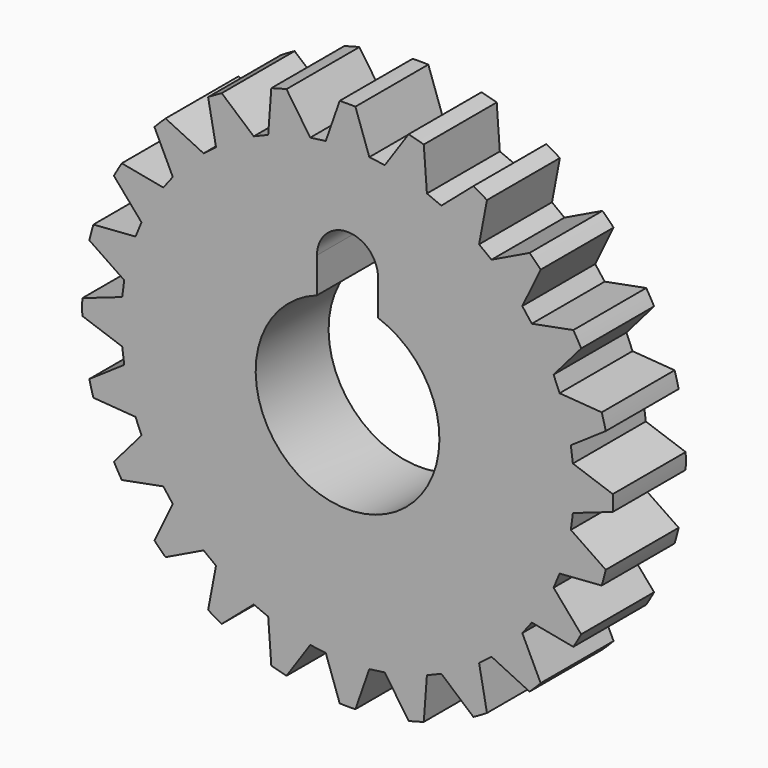
from build123d import *

# Parameters (mm, degrees)
F0_R            = 13.7922
F0_R_2          = 4.7752
F1_DEPTH        = 4.7371
F3_DEPTH        = 4.7381
F5_DEPTH        = 4.7381
F5_COPIES_COUNT = 24


# Not quite as in the source:
# - a pattern or mirror of a feature is missing from the dataset's text; its kind, count and spacing are read off the source's solid


with BuildPart() as f1:
    # F0 (on Front) → F1 (new body)
    with BuildSketch(Plane.XZ):
        Circle(F0_R)
        Circle(F0_R_2, mode=Mode.SUBTRACT)
    extrude(amount=F1_DEPTH)

    # F2 (on Front) → F3 (cut, through all)
    with BuildSketch(Plane.XZ):
        with BuildLine():
            Line((-1.5875, 6.3373), (-1.5875, 0))
            Line((-1.5875, 0), (1.5875, 0))
            Line((1.5875, 0), (1.5875, 6.3373))
            ThreePointArc((1.5875, 6.3373), (0, 7.9248), (-1.5875, 6.3373))
        make_face()
    extrude(amount=F3_DEPTH, mode=Mode.SUBTRACT)

    # F4 (on Front) → F5 (cut, through all)
    with BuildSketch(Plane.XZ):
        with BuildLine():
            Line((0.4064, 13.7922), (1.1320909341, 11.7126357032))
            Line((1.1320909341, 11.7126357032), (1.9379373174, 11.6065440142))
            Line((1.9379373174, 11.6065440142), (3.1771317781, 13.4274262413))
            ThreePointArc((3.1771317781, 13.4274262413), (1.8061892107, 13.7193691256), (0.4064, 13.7922))
        make_face()
    f5 = extrude(amount=F5_DEPTH, mode=Mode.SUBTRACT)

    # F5_copies: F5 ×24 about axis
    f5_copies_axis = Axis((0, 0, 0), (0, 1, 0))
    for i in range(1, F5_COPIES_COUNT):
        add(f5.rotate(f5_copies_axis, i * 360 / F5_COPIES_COUNT), mode=Mode.SUBTRACT)


solid = f1.part
